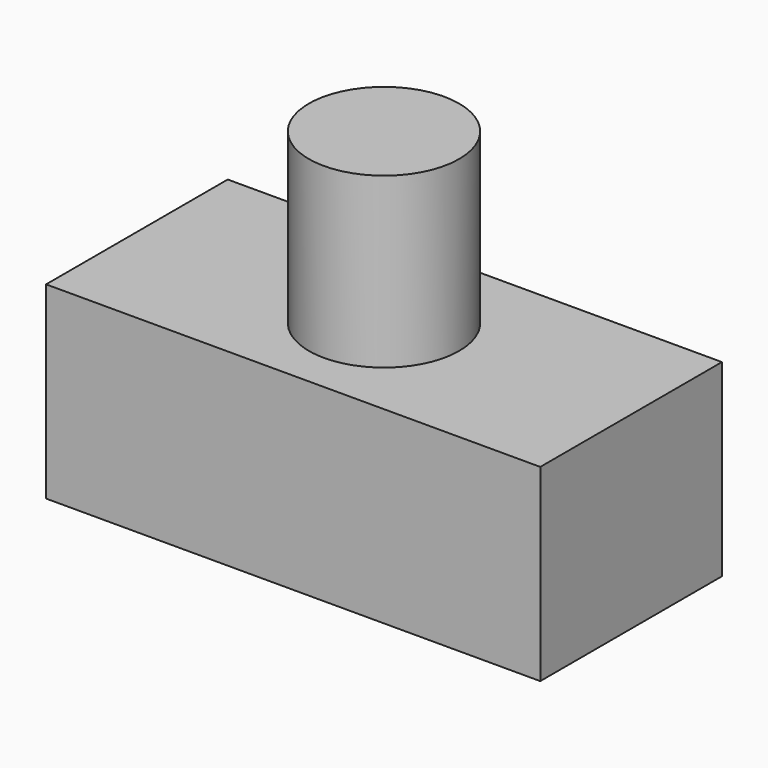
from build123d import *

# Parameters (mm, degrees)
F0_W         = 31.946439296
F0_H         = 14.6780936047
F1_DEPTH     = 12.192
F2_R         = 4.8571534919
F3_DEPTH     = 23.114
F4_TEXT_SIZE = 10.3929852937
F5_DEPTH     = 1.778


# Not quite as in the source:
# - Text() gives the source's letters only with a copy of the font that has no kerning and outlines rounded to 1/6400 em; it was checked with that copy


with BuildPart() as f1:
    # F0 (on Top) → F1 (new body)
    with BuildSketch(Plane.XY):
        Rectangle(F0_W, F0_H)
    extrude(amount=F1_DEPTH)

    # F2 (on Top) → F3 (join)
    with BuildSketch(Plane.XY):
        Circle(F2_R)
    extrude(amount=F3_DEPTH)

    # F4 (on Top) → F5 (join)
    with BuildSketch(Plane.XY):
        with Locations((-12.5195505098, -3.3097660635)):
            Text('Tiana', F4_TEXT_SIZE, font='Open Sans', font_style=FontStyle.ITALIC, text_align=(TextAlign.LEFT, TextAlign.BOTTOM))
    extrude(amount=-F5_DEPTH)


solid = f1.part
